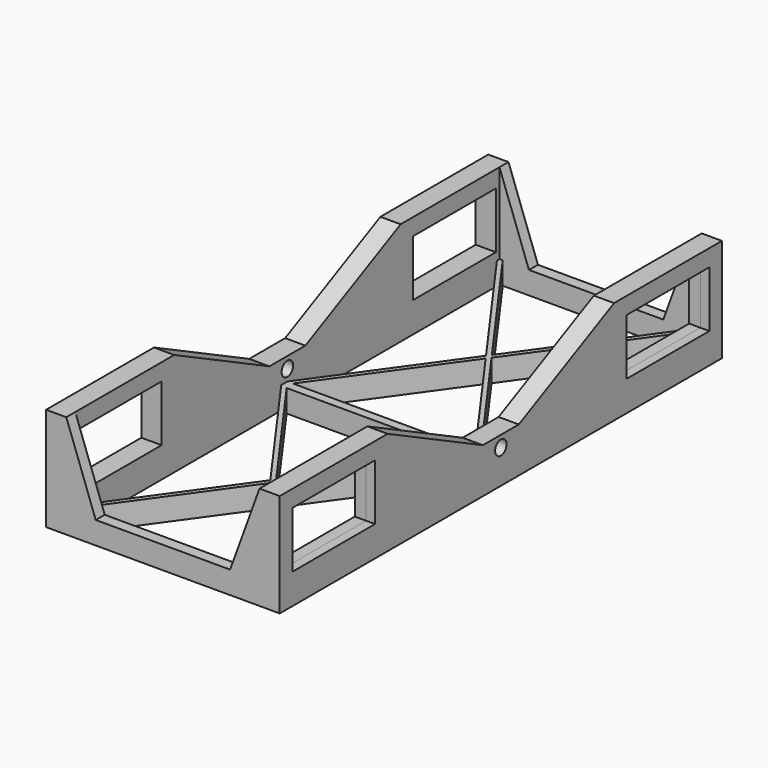
from build123d import *

# Parameters (mm, degrees)
F0_W       = 46
F0_H       = 123
F1_DEPTH   = 5
F2_W       = 30
F2_H       = 18
F3_DEPTH   = 46
F4_W       = 43
F4_H       = 30
F5_DEPTH   = 18
F6_W       = 23
F6_H       = 12.5
F7_DEPTH   = 46.001
F8_DEPTH   = 1
F9_DEPTH   = 1
F10_W      = 10
F10_H      = 10
F11_DEPTH  = 2.5
F12_W      = 10
F12_H      = 10
F13_DEPTH  = 2.5
F14_R      = 1.6
F15_DEPTH  = 48.001
F16_DEPTH  = 2
F10_W_2    = 23
F10_H_2    = 12.5
F11_FACE_W = 23
F11_FACE_H = 12.5
F11_FACE_R = 1.6
F17_DEPTH  = 2
F18_DEPTH  = 1
F19_DEPTH  = 1
F20_DEPTH  = 1
F22_DEPTH  = 2.5
F24_DEPTH  = 2.5
F26_DEPTH  = 4.5
F28_DEPTH  = 4.5


# Not quite as in the source:
# - after a boolean that leaves OpenCascade's solid faulty, fix() repairs it


with BuildPart() as f1:
    # F0 (on Top) → F1 (new body)
    with BuildSketch(Plane.XY):
        Rectangle(F0_W, F0_H)
        Polygon((-21.5, 60), (21.5, 60), (21.5, 58.2833176247), (21.5, 0), (21.5, -1), (21.5, -1.7166823753), (21.5, -60), (20.2697109644, -60), (-20.2697109644, -60), (-21.5, -60), (-21.5, -1.7166823753), (-21.5, -1), (-21.5, 0), (-21.5, 58.2833176247), align=None, mode=Mode.SUBTRACT)
        Polygon((0, 28.2833176247), (-0.6151445178, 29.1416588124), (-21.5, 0), (-20.2697109644, 0), align=None)
        Polygon((20.7833333333, -1), (21.5, 0), (20.2697109644, 0), (-20.2697109644, 0), (-21.5, 0), (-20.7833333333, -1), align=None)
        Polygon((-20.7833333333, -1), (-21.5, -1), (-21.5, -1.7166823753), (-0.6151445178, -30.8583411876), (0, -30), align=None)
        Polygon((21.5, -1.7166823753), (21.5, -1), (20.7833333333, -1), (0, -30), (0.6151445178, -30.8583411876), align=None)
        Polygon((0, -31.7166823753), (-0.6151445178, -30.8583411876), (-21.5, -60), (-20.2697109644, -60), align=None)
        Polygon((20.2697109644, -60), (21.5, -60), (0.6151445178, -30.8583411876), (0, -31.7166823753), align=None)
        Polygon((0.6151445178, -30.8583411876), (0, -30), (-0.6151445178, -30.8583411876), (0, -31.7166823753), align=None)
        Polygon((20.2697109644, 0), (21.5, 0), (0.6151445178, 29.1416588124), (0, 28.2833176247), align=None)
        Polygon((21.5, -1), (21.5, 0), (20.7833333333, -1), align=None)
        Polygon((-20.7833333333, -1), (-21.5, 0), (-21.5, -1), align=None)
        Polygon((0.6151445178, 29.1416588124), (0, 30), (-0.6151445178, 29.1416588124), (0, 28.2833176247), align=None)
        Polygon((21.5, 58.2833176247), (21.5, 60), (0, 30), (0.6151445178, 29.1416588124), align=None)
        Polygon((0, 30), (-21.5, 60), (-21.5, 58.2833176247), (-0.6151445178, 29.1416588124), align=None)
    extrude(amount=F1_DEPTH)

    # F2 (on face) → F3 (join)
    with BuildSketch(Plane(origin=(-23, 0, 0), x_dir=(0, -1, 0), z_dir=(-1, 0, 0))):
        with Locations((-46.5, 14)):
            Rectangle(F2_W, F2_H)
        with Locations((46.5, 14)):
            Rectangle(F2_W, F2_H)
    extrude(amount=-F3_DEPTH)

    # F4 (on face) → F5 (cut)
    with BuildSketch(Plane.XY.offset(23)):
        with Locations((0, 46.5)):
            Rectangle(F4_W, F4_H)
        with Locations((0, -46.5)):
            Rectangle(F4_W, F4_H)
    extrude(amount=-F5_DEPTH, mode=Mode.SUBTRACT)

    # F6 (on face) → F7 (cut, through all)
    with BuildSketch(Plane(origin=(-23, 0, 0), x_dir=(0, -1, 0), z_dir=(-1, 0, 0))):
        with Locations((-46.5, 13)):
            Rectangle(F6_W, F6_H)
        with Locations((46.5, 13)):
            Rectangle(F6_W, F6_H)
    extrude(amount=-F7_DEPTH, mode=Mode.SUBTRACT)

    # F8 (add): a face of the model
    f8_faces = [f1.faces().sort_by_distance(p)[0] for p in [
        (-23, 60.2486806962, 11.5),
    ]]
    extrude(f8_faces, amount=F8_DEPTH)

    # F9 (add): a face of the model
    f9_faces = [f1.faces().sort_by_distance(p)[0] for p in [
        (23, -60.2486806962, 11.5),
    ]]
    extrude(f9_faces, amount=F9_DEPTH)

    # F10 (on face) → F11 (join)
    with BuildSketch(Plane(origin=(-24, 0, 0), x_dir=(0, -1, 0), z_dir=(-1, 0, 0))):
        with Locations((0, 5)):
            Rectangle(F10_W, F10_H)
    extrude(amount=-F11_DEPTH)

    # F12 (on face) → F13 (join)
    with BuildSketch(Plane.YZ.offset(24)):
        with Locations((0, 5)):
            Rectangle(F12_W, F12_H)
    extrude(amount=-F13_DEPTH)

    # F14 (on face) → F15 (cut, through all)
    with BuildSketch(Plane.YZ.offset(24)):
        with Locations((0, 7.5)):
            Circle(F14_R)
    extrude(amount=-F15_DEPTH, mode=Mode.SUBTRACT)

    # F16 (add): a face of the model
    f16_faces = [f1.faces().sort_by_distance(p)[0] for p in [
        (24, 0, 1.2513193038),
    ]]
    extrude(f16_faces, amount=F16_DEPTH)

    # F10 (on face) + F11_face (on face) → F17 (join)
    with BuildSketch(Plane(origin=(-24, 0, 0), x_dir=(0, -1, 0), z_dir=(-1, 0, 0))):
        Polygon((-61.5, 0), (-5, 0), (-5, 5), (-31.5, 5), (-31.5, 23), (-61.5, 23), align=None)
        with Locations((-46.5, 13)):
            Rectangle(F10_W_2, F10_H_2, mode=Mode.SUBTRACT)
    with BuildSketch(Plane(origin=(-24, 0, 8.1734325349), x_dir=(0, -1, 0), z_dir=(-1, 0, 0))):
        Polygon((-61.5, -8.1734325349), (61.5, -8.1734325349), (61.5, 14.8265674651), (31.5, 14.8265674651), (31.5, -3.1734325349), (5, -3.1734325349), (5, 1.8265674651), (-5, 1.8265674651), (-5, -3.1734325349), (-31.5, -3.1734325349), (-31.5, 14.8265674651), (-61.5, 14.8265674651), align=None)
        with Locations((-46.5, 4.8265674651)):
            Rectangle(F11_FACE_W, F11_FACE_H, mode=Mode.SUBTRACT)
        with Locations((46.5, 4.8265674651)):
            Rectangle(F11_FACE_W, F11_FACE_H, mode=Mode.SUBTRACT)
        with Locations((0, -0.6734325349)):
            Circle(F11_FACE_R, mode=Mode.SUBTRACT)
    extrude(amount=F17_DEPTH)

    # F18 (add): a face of the model
    f18_faces = [f1.faces().sort_by_distance(p)[0] for p in [
        (0, 60, 2.5),
    ]]
    extrude(f18_faces, amount=F18_DEPTH)

    add(f1.part.fix(), mode=Mode.REPLACE)

    # F19 (add): a face of the model
    f19_faces = [f1.faces().sort_by_distance(p)[0] for p in [
        (0, -60, 2.5),
    ]]
    extrude(f19_faces, amount=F19_DEPTH)

    # F20 (add): a face of the model
    f20_faces = [f1.faces().sort_by_distance(p)[0] for p in [
        (0, -1, 2.5),
    ]]
    extrude(f20_faces, amount=F20_DEPTH)

    # F21 (on face) → F22 (join)
    with BuildSketch(Plane(origin=(0, 61.5, 0), x_dir=(-1, 0, 0), z_dir=(0, 1, 0))):
        Polygon((-21.5, 23), (-21.5, 5), (-14.9485357832, 5), align=None)
        Polygon((21.5, 23), (14.9485357832, 5), (21.5, 5), align=None)
    extrude(amount=-F22_DEPTH)

    add(f1.part.fix(), mode=Mode.REPLACE)

    # F23 (on face) → F24 (join)
    with BuildSketch(Plane.XZ.offset(61.5)):
        Polygon((21.5, 23), (14.9485357832, 5), (21.5, 5), align=None)
        Polygon((-14.9485357832, 5), (-21.5, 23), (-21.5, 5), align=None)
    extrude(amount=-F24_DEPTH)

    # F25 (on face) → F26 (join)
    with BuildSketch(Plane(origin=(-26, 0, 0), x_dir=(0, -1, 0), z_dir=(-1, 0, 0))):
        Polygon((-5, 10), (-31.5, 23), (-31.5, 5), (-5, 5), align=None)
        Polygon((31.5, 23), (5, 10), (5, 5), (31.5, 5), align=None)
    extrude(amount=-F26_DEPTH)

    # F27 (on face) → F28 (join)
    with BuildSketch(Plane.YZ.offset(26)):
        Polygon((31.5, 5), (31.5, 23), (5, 10), (5, 5), align=None)
        Polygon((-5, 5), (-5, 10), (-31.5, 23), (-31.5, 5), align=None)
    extrude(amount=-F28_DEPTH)


solid = f1.part
